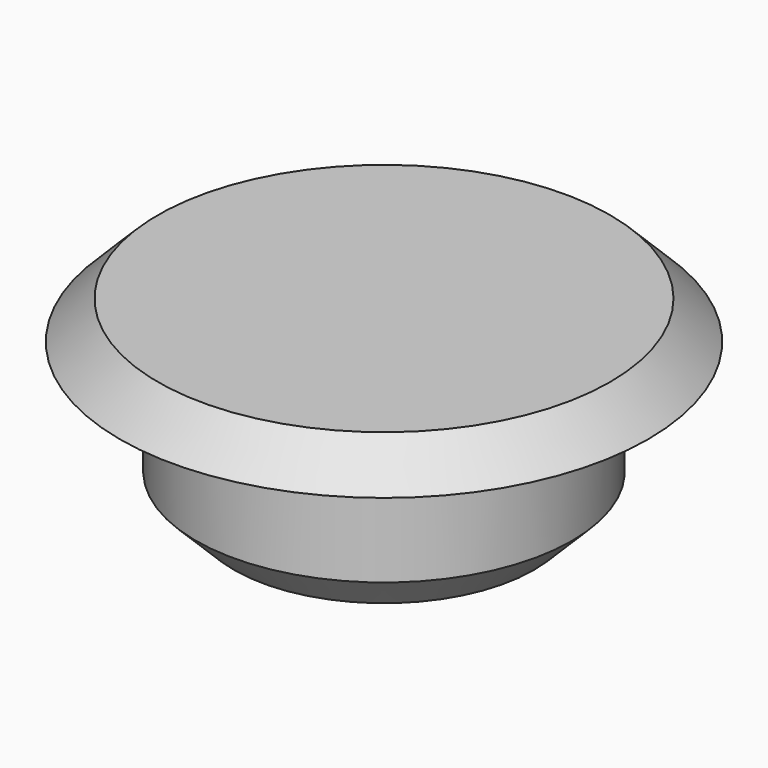
from build123d import *

# Parameters (mm, degrees)
F0_R        = 4.945
F0_R_2      = 3.445
F1_DEPTH    = 4
F0_R_3      = 6.945
F1_FACE_R   = 4.945
F1_FACE_R_2 = 3.445
F2_DEPTH    = 1
F3_SIZE     = 0.99999
F4_SIZE2    = 1
F4_SIZE     = 1


# Not quite as in the source:
# - a fillet or chamfer is up to 0.001 mm smaller than in the source, because OpenCascade refuses the exact size


with BuildPart() as f1:
    # F0 (on Top) → F1 (new body)
    with BuildSketch(Plane.XY):
        Circle(F0_R)
        Circle(F0_R_2, mode=Mode.SUBTRACT)
    extrude(amount=-F1_DEPTH)

    # F0 (on Top) + F1_face (on face) → F2 (join)
    with BuildSketch(Plane.XY):
        Circle(F0_R_3)
        Circle(F0_R, mode=Mode.SUBTRACT)
        Circle(F0_R_2)
    with BuildSketch(Plane.XY):
        Circle(F1_FACE_R)
        Circle(F1_FACE_R_2, mode=Mode.SUBTRACT)
    extrude(amount=F2_DEPTH)

    # F3 (size 1 in the source; OpenCascade refuses exactly that, so slightly less here)
    f3_edges = [f1.edges().sort_by_distance(p)[0] for p in [
        (-6.945, 0, 1),
    ]]
    chamfer(f3_edges, length=F3_SIZE)

    # F4
    f4_edges = [f1.edges().sort_by_distance(p)[0] for p in [
        (-4.945, 0, -4),
    ]]
    chamfer(f4_edges, length=F4_SIZE, length2=F4_SIZE2)


solid = f1.part
